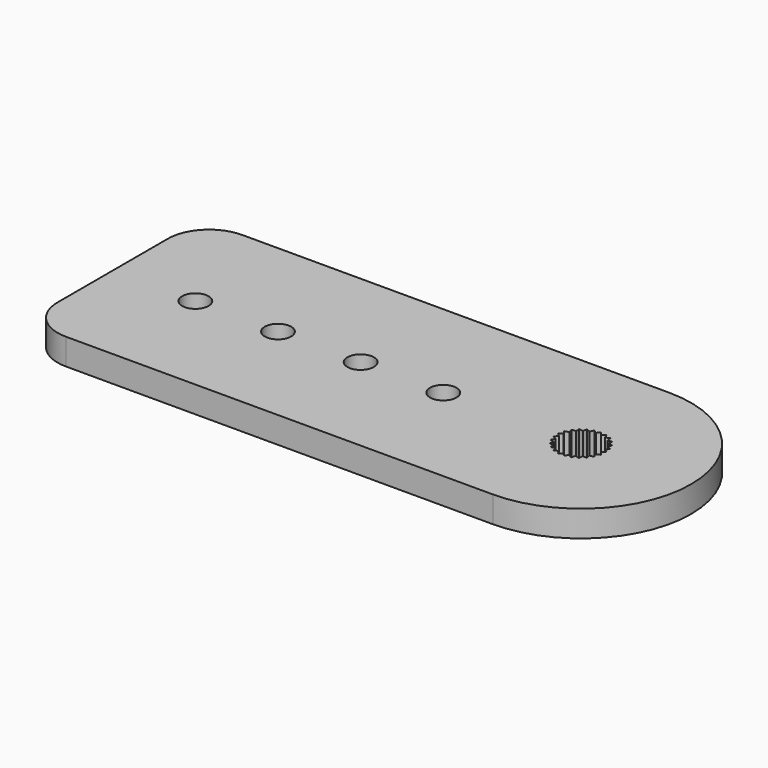
from build123d import *

# Parameters (mm, degrees)
F0_R     = 1.6
F1_DEPTH = 3.175


with BuildPart() as f1:
    # F0 (on Top) → F1 (new body)
    with BuildSketch(Plane.XY):
        with BuildLine():
            Line((-51.6649944294, -13.3350055706), (0, -13.3350055706))
            ThreePointArc((0, -13.3350055706), (13.3350055706, 0), (0, 13.3350055706))
            Line((0, 13.3350055706), (-51.6649944294, 13.3350055706))
            ThreePointArc((-51.6649944294, 13.3350055706), (-55.2005283353, 11.8705394766), (-56.6649944294, 8.3350055706))
            Line((-56.6649944294, 8.3350055706), (-56.6649944294, -8.3350055706))
            ThreePointArc((-56.6649944294, -8.3350055706), (-55.2005283353, -11.8705394766), (-51.6649944294, -13.3350055706))
        make_face()
        with Locations((-46.6649944294, 0)):
            Circle(F0_R, mode=Mode.SUBTRACT)
        with Locations((-36.6649944294, 0)):
            Circle(F0_R, mode=Mode.SUBTRACT)
        with Locations((-26.6649944294, 0)):
            Circle(F0_R, mode=Mode.SUBTRACT)
        with Locations((-16.6649944294, 0)):
            Circle(F0_R, mode=Mode.SUBTRACT)
        Polygon((-2.3131272616, 1.150841372), (-2.4811892868, 1.651717782), (-1.9542535042, 1.6899369317), (-1.992472654, 2.2168727143), (-1.4725868119, 2.1228475389), (-1.3785616365, 2.6427333809), (-0.8983920744, 2.4223718279), (-0.6780305213, 2.90254139), (-0.2677480588, 2.5696895861), (0.0651037451, 2.9799720486), (0.379719552, 2.555544297), (0.8041473037, 2.8701601039), (1.0033279869, 2.380824761), (1.4926633298, 2.5800054442), (1.5638936344, 2.0565092492), (2.0873898293, 2.1277395538), (2.0261940932, 1.6029756981), (2.5509579489, 1.5417799619), (2.3611813253, 1.0487212884), (2.8542399989, 0.8589446648), (2.547806851, 0.4285718633), (2.9781796525, 0.1221387154), (2.574344302, -0.2185063082), (2.9149893256, -0.6223416587), (2.4391262327, -0.8518549247), (2.6686394987, -1.3277180175), (2.1506488918, -1.4316783634), (2.2546092377, -1.9496689703), (1.7270383715, -1.9215441851), (1.6989135863, -2.4491150513), (1.1949116786, -2.2906723188), (1.0364689461, -2.7946742265), (0.5877042905, -2.5158690862), (0.3088991502, -2.9646337418), (-0.0564307197, -2.5829845462), (-0.4380799154, -2.9483144161), (-0.6970199802, -2.4878015876), (-1.1575328087, -2.7467416524), (-1.2938129119, -2.2363009057), (-1.8042536586, -2.3725810089), (-1.80931082, -1.8442852134), (-2.3376066155, -1.8493423749), (-2.2111230752, -1.3363862984), (-2.7240791517, -1.209902758), (-2.4740023355, -0.7445173173), (-2.9393877762, -0.4944405012), (-2.5814309304, -0.105867575), (-2.9700038565, 0.2520892708), (-2.5266587261, 0.5394342163), (-2.8140036716, 0.9827793468), align=None, mode=Mode.SUBTRACT)
    extrude(amount=F1_DEPTH)


solid = f1.part
